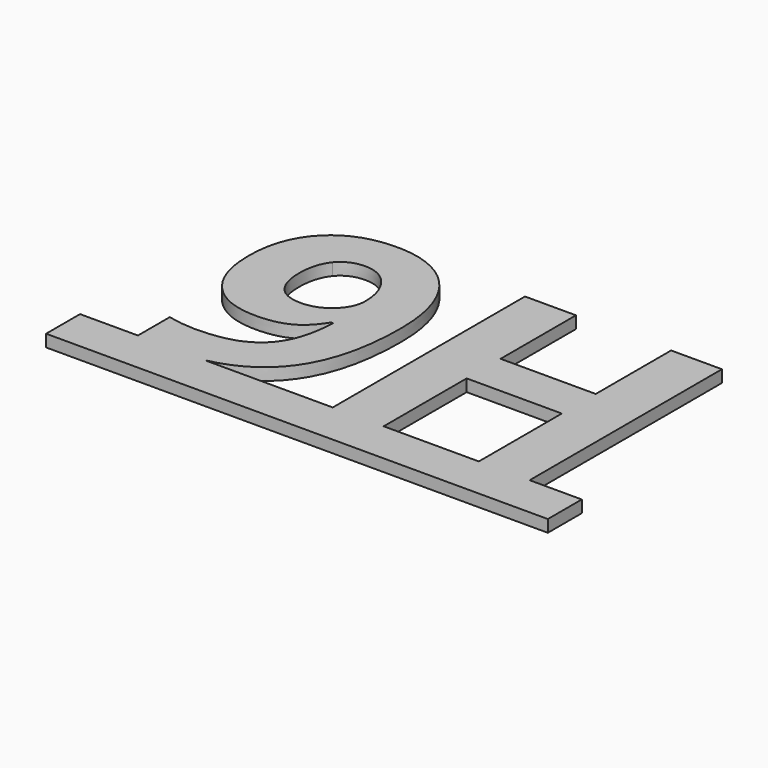
from build123d import *

# Parameters (mm, degrees)
F1_DEPTH = 50.8


# Not quite as in the source:
# - a feature names something its author has since deleted; it is built from what else it names


with BuildPart() as f1:
    # F0 (on Top) → F1 (new body)
    with BuildSketch(Plane.XY):
        with BuildLine():
            Line((-428.8131256104, -528.4897685051), (-428.8131256104, -706.2897685051))
            Line((-428.8131256104, -706.2897685051), (1674.4038882785, -706.2897685051))
            Line((1674.4038882785, -706.2897685051), (1674.4038882785, -528.4897685051))
            Line((1674.4038882785, -528.4897685051), (1455.9021521674, -528.4897685051))
            Line((1455.9021521674, -528.4897685051), (1242.9125688341, -528.4897685051))
            Line((1242.9125688341, -528.4897685051), (844.0531938341, -528.4897685051))
            Line((844.0531938341, -528.4897685051), (630.4021521674, -528.4897685051))
            Line((630.4021521674, -528.4897685051), (93.9480274003, -528.4897685051))
            add(Edge.make_bspline(
                [(93.9480274003, -528.4897685051), (27.9501754164, -542.3803935051), (-50.2384728326, -542.3803935051)],
                knots=[0.6924376574, 0.6924376574, 0.6924376574, 1, 1, 1], degree=2))
            add(Edge.make_bspline(
                [(-50.2384728326, -542.3803935051), (-139.9763200548, -542.3803935051), (-186.057917277, -532.6790046162)],
                knots=[0, 0, 0, 1, 1, 1], degree=2))
            Line((-186.057917277, -532.6790046162), (-186.057917277, -528.4897685051))
            Line((-186.057917277, -528.4897685051), (-428.8131256104, -528.4897685051))
        make_face()
        Polygon((1242.9125688341, -528.4897685051), (1455.9021521674, -528.4897685051), (1455.9021521674, 478.9112731616), (1242.9125688341, 478.9112731616), (1242.9125688341, 84.0206481616), (844.0531938341, 84.0206481616), (844.0531938341, 478.9112731616), (630.4021521674, 478.9112731616), (630.4021521674, -528.4897685051), (844.0531938341, -528.4897685051), (844.0531938341, -93.691157394), (1242.9125688341, -93.691157394), align=None)
        with BuildLine():
            Line((-186.057917277, -361.8022685051), (-186.057917277, -528.4897685051))
            Line((-186.057917277, -528.4897685051), (93.9480274003, -528.4897685051))
            add(Edge.make_bspline(
                [(329.3283674452, -395.5366435051), (242.5338316042, -497.2167857568), (93.9480274003, -528.4897685051)],
                knots=[0, 0, 0, 0.6924376574, 0.6924376574, 0.6924376574], degree=2))
            add(Edge.make_bspline(
                [(454.6747216119, 48.9633564949), (454.6747216119, -248.6928935051), (329.3283674452, -395.5366435051)],
                knots=[0, 0, 0, 1, 1, 1], degree=2))
            add(Edge.make_bspline(
                [(409.9160410563, 286.316655106), (454.6747216119, 186.7671759393), (454.6747216119, 48.9633564949)],
                knots=[0, 0, 0, 1, 1, 1], degree=2))
            add(Edge.make_bspline(
                [(281.4828813341, 438.2315856616), (365.1573605008, 385.8661342727), (409.9160410563, 286.316655106)],
                knots=[0, 0, 0, 1, 1, 1], degree=2))
            add(Edge.make_bspline(
                [(86.0219438341, 490.5970370505), (197.8084021674, 490.5970370505), (281.4828813341, 438.2315856616)],
                knots=[0, 0, 0, 1, 1, 1], degree=2))
            add(Edge.make_bspline(
                [(-164.3400353326, 396.5597106616), (-72.2870839437, 490.5970370505), (86.0219438341, 490.5970370505)],
                knots=[0, 0, 0, 1, 1, 1], degree=2))
            add(Edge.make_bspline(
                [(-256.3929867215, 140.465092606), (-256.3929867215, 302.5223842727), (-164.3400353326, 396.5597106616)],
                knots=[0, 0, 0, 1, 1, 1], degree=2))
            add(Edge.make_bspline(
                [(-180.5457644992, -94.0218865607), (-256.3929867215, -9.6859490607), (-256.3929867215, 140.465092606)],
                knots=[0, 0, 0, 1, 1, 1], degree=2))
            add(Edge.make_bspline(
                [(26.9316660563, -178.3578240607), (-104.698542277, -178.3578240607), (-180.5457644992, -94.0218865607)],
                knots=[0, 0, 0, 1, 1, 1], degree=2))
            add(Edge.make_bspline(
                [(157.7901730008, -152.230219894), (105.4247216119, -178.3578240607), (26.9316660563, -178.3578240607)],
                knots=[0, 0, 0, 1, 1, 1], degree=2))
            add(Edge.make_bspline(
                [(250.0636105008, -61.2796990607), (210.1556243896, -126.1026157273), (157.7901730008, -152.230219894)],
                knots=[0, 0, 0, 1, 1, 1], degree=2))
            Line((250.0636105008, -61.2796990607), (258.442082723, -61.2796990607))
            add(Edge.make_bspline(
                [(216.3292355008, -246.3777893384), (252.9299299452, -179.2397685051), (258.442082723, -61.2796990607)],
                knots=[0, 0, 0, 1, 1, 1], degree=2))
            add(Edge.make_bspline(
                [(110.8266313341, -344.8248379495), (179.7285410563, -313.5158101718), (216.3292355008, -246.3777893384)],
                knots=[0, 0, 0, 1, 1, 1], degree=2))
            add(Edge.make_bspline(
                [(-64.7905561659, -376.1338657273), (41.9247216119, -376.1338657273), (110.8266313341, -344.8248379495)],
                knots=[0, 0, 0, 1, 1, 1], degree=2))
            add(Edge.make_bspline(
                [(-186.057917277, -361.8022685051), (-128.0700700548, -376.1338657273), (-64.7905561659, -376.1338657273)],
                knots=[0, 0, 0, 1, 1, 1], degree=2))
        make_face()
        with BuildLine():
            add(Edge.make_bspline(
                [(90.2111799452, 319.7203009393), (24.0653466119, 319.7203009393), (-13.0865631104, 274.1899189949)],
                knots=[0, 0, 0, 1, 1, 1], degree=2))
            add(Edge.make_bspline(
                [(200.1235063341, 263.1656134393), (157.0184716119, 319.7203009393), (90.2111799452, 319.7203009393)],
                knots=[0, 0, 0, 1, 1, 1], degree=2))
            add(Edge.make_bspline(
                [(243.2285410563, 124.8105787171), (243.2285410563, 206.6109259393), (200.1235063341, 263.1656134393)],
                knots=[0, 0, 0, 1, 1, 1], degree=2))
            add(Edge.make_bspline(
                [(197.0367007785, 27.2454745505), (243.2285410563, 69.6890509393), (243.2285410563, 124.8105787171)],
                knots=[0, 0, 0, 1, 1, 1], degree=2))
            add(Edge.make_bspline(
                [(86.0219438341, -15.1981018384), (150.8448605008, -15.1981018384), (197.0367007785, 27.2454745505)],
                knots=[0, 0, 0, 1, 1, 1], degree=2))
            add(Edge.make_bspline(
                [(-16.5040978326, 27.5762037171), (17.2302771674, -15.1981018384), (86.0219438341, -15.1981018384)],
                knots=[0, 0, 0, 1, 1, 1], degree=2))
            add(Edge.make_bspline(
                [(-50.2384728326, 143.3314120505), (-50.2384728326, 70.3505092727), (-16.5040978326, 27.5762037171)],
                knots=[0, 0, 0, 1, 1, 1], degree=2))
            add(Edge.make_bspline(
                [(-13.0865631104, 274.1899189949), (-50.2384728326, 228.6595370505), (-50.2384728326, 143.3314120505)],
                knots=[0, 0, 0, 1, 1, 1], degree=2))
        make_face(mode=Mode.SUBTRACT)
        with BuildLine():
            Line((93.9480274003, -528.4897685051), (-186.057917277, -528.4897685051))
            Line((-186.057917277, -528.4897685051), (-186.057917277, -532.6790046162))
            add(Edge.make_bspline(
                [(-50.2384728326, -542.3803935051), (-139.9763200548, -542.3803935051), (-186.057917277, -532.6790046162)],
                knots=[0, 0, 0, 1, 1, 1], degree=2))
            add(Edge.make_bspline(
                [(93.9480274003, -528.4897685051), (27.9501754164, -542.3803935051), (-50.2384728326, -542.3803935051)],
                knots=[0.6924376574, 0.6924376574, 0.6924376574, 1, 1, 1], degree=2))
        make_face()
    extrude(amount=F1_DEPTH)


solid = f1.part
